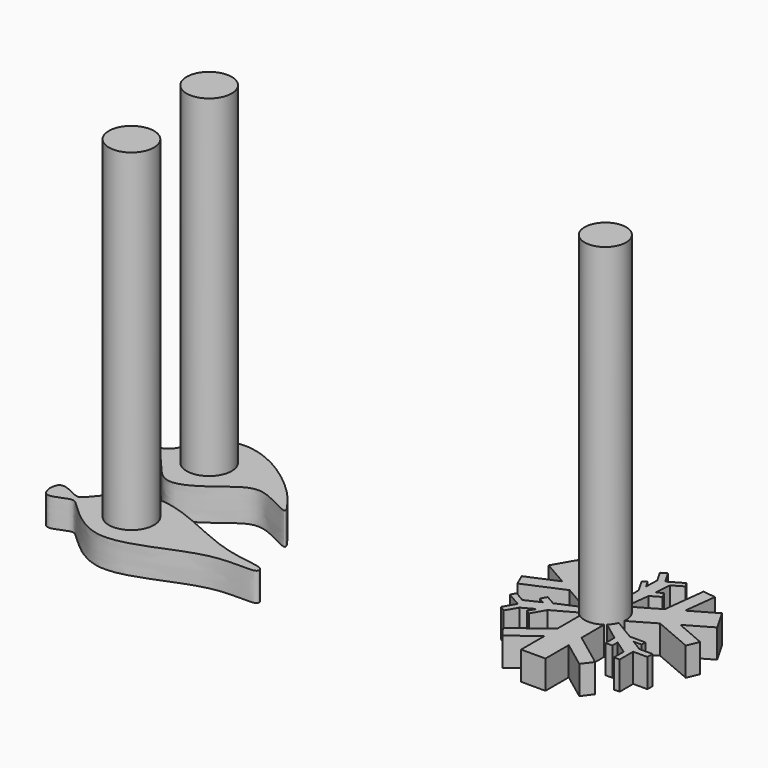
from build123d import *

# Parameters (mm, degrees)
F2_DEPTH  = 2
F1_R      = 1.4605
F3_DEPTH  = 25.4
F5_DEPTH  = 1
F7_SCALE  = 2.25
F9_R      = 1.5875
F10_DEPTH = 25.4
F13_DEPTH = 2
F12_R     = 1.5875
F14_DEPTH = 25.4


# Not quite as in the source:
# - ends of sketch curves that miss each other by under 0.0002 mm in the source are joined
# - a feature names something its author has since deleted; it is built from what else it names


with BuildPart() as f2:
    # F0 (on Top) → F2 (new body)
    with BuildSketch(Plane.XY):
        Polygon((0.3471141813, -0.6012196677), (-0.1371353539, -0.2375256701), (-0.2495522491, -0.4322374442), (-0.4318002417, -0.747900227), (-0.6211034032, -0.6386059958), (-0.8508992831, -0.7662402189), (-0.8508992831, -3.1749998652), (-0.8508992831, -4.3027643429), (-0.8508992831, -6.3499998652), (0.8636007169, -6.3499998652), (0.8636007169, -4.3027643429), (0.8636007169, -3.1749998652), (0.8636007169, -0.9891251569), (0.483299174, -0.703500952), (0.4254495248, -0.7369004626), align=None)
        Polygon((-0.8508992831, -4.3027643429), (-0.8508992831, -3.1749998652), (-3.2412230885, -4.9631580294), (-2.7002857532, -5.6862570345), align=None)
        Polygon((3.2539245223, -4.9631580294), (0.8636007169, -3.1749998652), (0.8636007169, -4.3027643429), (2.7129871871, -5.6862570345), align=None)
        Polygon((-0.8508992831, -0.0667988863), (-0.6942285962, 1.348e-07), (-0.8508992831, 1.348e-07), align=None)
        Polygon((-0.6942285962, 1.348e-07), (-0.1371355874, 0.2375255353), (-0.2495524826, 0.4322373094), (-0.4318004752, 0.7479000922), (-0.2424973138, 0.8571943234), (-0.2381338534, 1.1200205046), (-2.3241808987, 2.3244003278), (-3.3008535859, 2.8882825667), (-5.0738115558, 3.9119003278), (-5.9310615558, 2.427099773), (-4.1581035859, 1.4034820119), (-3.1814308987, 0.839599773), (-1.2884078719, -0.2533375811), (-0.8508992831, -0.0667988863), (-0.8508992831, 1.348e-07), align=None)
        Polygon((-0.8508992831, -0.7662402189), (-0.8508992831, -0.5059332827), (-1.2884078719, -0.2533375811), (-2.9236705151, -0.950557629), (-3.6042041051, -0.5576513776), (-3.8423290847, -0.9700959409), (-3.4298843198, -1.208221037), (-4.4835569455, -1.6997353006), (-5.2259572804, -1.2711102674), (-5.4283635946, -1.6216882874), (-4.3972519847, -2.2170008529), (-4.8973144653, -3.0831344762), (-4.5054921503, -3.3093531953), (-4.0411482187, -2.5050859137), (-3.2032690115, -2.0539615173), (-3.4890190337, -2.5488950739), (-3.2003078595, -2.7155825481), (-2.6526203364, -1.7669599314), align=None)
        Polygon((-5.9251831976, -0.3364022836), (-3.1814308987, 0.839599773), (-4.1581035859, 1.4034820119), (-6.2809366379, 0.4936126931), align=None)
        Polygon((-3.3008535859, 2.8882825667), (-2.3241808987, 2.3244003278), (-2.6776093922, 5.2885605486), (-3.5743001677, 5.181644577), align=None)
        Polygon((-0.0127014339, 0.9898670365), (0.4248071549, 1.242462738), (0.6386282031, 3.0072517529), (1.3191617931, 3.4001580042), (1.0810368134, 3.8126025675), (0.6685920485, 3.5744774715), (0.7697645227, 4.7327418644), (1.5121648577, 5.1613668976), (1.3097585434, 5.5119449176), (0.2786469335, 4.916632352), (-0.2214155471, 5.7827659754), (-0.6132378621, 5.5565472563), (-0.1488939305, 4.7522799747), (-0.1771483466, 3.8010930978), (-0.4628983688, 4.2960266544), (-0.7516095429, 4.1293391803), (-0.2039220199, 3.1807165637), (-0.2381338534, 1.1200205046), align=None)
        Polygon((2.6712586753, 5.299560313), (2.3178301818, 2.3354000922), (3.294502869, 2.8992823311), (3.5679494508, 5.1926443415), align=None)
        Polygon((0.2742709413, 1.348e-07), (0.4991047317, 1.348e-07), (0.8636007169, 1.348e-07), (0.8636007169, -0.2185883276), (1.0890331365, -0.3537802858), (3.1750801818, 0.8505995374), (4.151752869, 1.4144817763), (5.9247108388, 2.4380995374), (5.0674608388, 3.9229000922), (3.294502869, 2.8992823311), (2.3178301818, 2.3354000922), (0.4248071549, 1.242462738), (0.3676001091, 0.7702998383), (0.4254497583, 0.7369003278), (0.3471144148, 0.6012195329), align=None)
        Polygon((4.151752869, 1.4144817763), (3.1750801818, 0.8505995374), (5.9188324807, -0.3254025192), (6.274585921, 0.5046124575), align=None)
        Polygon((1.0890331365, -0.3537802858), (0.8636007169, -0.4839337539), (0.8636007169, -0.9891251569), (2.285042312, -2.0566941239), (2.285042312, -2.8425066266), (2.7612922713, -2.8425066266), (2.7612922713, -2.3662564345), (3.7137924228, -3.0330065638), (3.7137924228, -3.8902566303), (4.1186050512, -3.8902566303), (4.1186050512, -2.6996314991), (5.1187300123, -2.6996314991), (5.1187300123, -2.2471940611), (4.1900421493, -2.2471940611), (3.3804173581, -1.7471315805), (3.9519174024, -1.7471315805), (3.9519174024, -1.4137566322), (2.8565423563, -1.4137566322), align=None)
        Polygon((0.8636007169, -0.2185883276), (0.4991047317, 1.348e-07), (0.2742709413, 1.348e-07), (0.2266974185, -0.3926517164), (0.3471141813, -0.6012196677), (0.483299174, -0.703500952), (0.8636007169, -0.4839337539), align=None)
        Polygon((-0.1371353539, -0.2375256701), (-0.4533950705, 1.348e-07), (-0.6942285962, 1.348e-07), (-0.8508992831, -0.0667988863), (-0.8508992831, -0.5059332827), (-0.6211034032, -0.6386059958), (-0.2495522491, -0.4322374442), align=None)
        Polygon((0.226697652, 0.3926515816), (0.3471144148, 0.6012195329), (0.3676001091, 0.7702998383), (-0.0127014339, 0.9898670365), (-0.2424973138, 0.8571943234), (-0.2495524826, 0.4322373094), (-0.1371355874, 0.2375255353), align=None)
        Polygon((-0.0127014339, 0.9898670365), (0.3676001091, 0.7702998383), (0.4248071549, 1.242462738), align=None)
        Polygon((1.0890331365, -0.3537802858), (0.8636007169, -0.2185883276), (0.8636007169, -0.4839337539), align=None)
        Polygon((-0.4318002417, -0.747900227), (-0.2495522491, -0.4322374442), (-0.6211034032, -0.6386059958), align=None)
        Polygon((-0.8508992831, -0.7662402189), (-0.6211034032, -0.6386059958), (-0.8508992831, -0.5059332827), align=None)
        Polygon((-0.4318004752, 0.7479000922), (-0.2495524826, 0.4322373094), (-0.2424973138, 0.8571943234), align=None)
        Polygon((-0.2424973138, 0.8571943234), (-0.0127014339, 0.9898670365), (-0.2381338534, 1.1200205046), align=None)
        Polygon((0, 1.348e-07), (0.2742709413, 1.348e-07), (0.3471144148, 0.6012195329), (0.226697652, 0.3926515816), align=None)
        Polygon((-0.1371355874, 0.2375255353), (-1.167e-07, -6.74e-08), (0.226697652, 0.3926515816), align=None)
        Polygon((-0.4533950705, 1.348e-07), (0, 1.348e-07), (-0.1371355874, 0.2375255353), (-0.6942285962, 1.348e-07), align=None)
        Polygon((-0.1371353539, -0.2375256701), (1.167e-07, -6.74e-08), (-0.4533950705, 1.348e-07), align=None)
        Polygon((0.2266974185, -0.3926517164), (-1.167e-07, -6.74e-08), (-0.1371353539, -0.2375256701), (0.3471141813, -0.6012196677), align=None)
        Polygon((0.2266974185, -0.3926517164), (0.2742709413, 1.348e-07), (0, 1.348e-07), align=None)
        Polygon((0.3676001091, 0.7702998383), (0.3471144148, 0.6012195329), (0.4254497583, 0.7369003278), align=None)
        Polygon((0.483299174, -0.703500952), (0.3471141813, -0.6012196677), (0.4254495248, -0.7369004626), align=None)
    extrude(amount=F2_DEPTH)

    # F1 (on Top) → F3 (join)
    with BuildSketch(Plane.XY):
        Circle(F1_R)
    extrude(amount=F3_DEPTH)


with BuildPart() as f5:
    # F4 (on Top) → F5 (new body)
    with BuildSketch(Plane.XY):
        with BuildLine():
            add(Edge.make_bspline(
                [(-29.8669375479, 0.2857499931), (-29.7440304745, 0.3571436979), (-29.1547614666, -0.031081706), (-28.6573535606, 1.9086215428), (-26.8097076406, 1.4876465764), (-25.6137182394, 0.4424417951), (-25.3000873709, 0.0757578444), (-24.7765698555, -0.6160305024), (-25.5747691832, -0.1631625611), (-26.2801418295, 0.1338939544), (-26.9852315195, -0.4157522042), (-28.4156101147, -1.4829106615), (-29.1578723902, 0.3232844338), (-30.049192476, -0.1925589818), (-29.9590967439, 0.2322169762), (-29.8669375479, 0.2857499931)],
                knots=[0, 0, 0, 0, 0.0595602967, 0.1590621278, 0.2623182491, 0.3653254409, 0.4276419031, 0.4859643703, 0.5478739218, 0.6200200353, 0.696962825, 0.7939279281, 0.8918484857, 0.9553400069, 1, 1, 1, 1], degree=3))
        make_face()
    extrude(amount=F5_DEPTH)


with BuildPart() as f5_1:
    # F7: moved
    add(f5.part.scale(F7_SCALE).moved(Location((34.892889671, -0.5655468703, -1.25))))


with BuildPart() as f5_2:
    # F8: moved
    add(f5_1.part.moved(Location((0, 0, 1))))

    # F9 (on Top) → F10 (join)
    with BuildSketch(Plane.XY):
        with Locations((-28.1345900148, 0.302218803)):
            Circle(F9_R)
    extrude(amount=F10_DEPTH)


with BuildPart() as f13:
    # F11 (on Top) → F13 (new body)
    with BuildSketch(Plane.XY):
        with BuildLine():
            add(Edge.make_bspline(
                [(-32.8794009984, -6.9053298794), (-32.5540037989, -6.6793889467), (-31.3817308567, -7.5046151757), (-30.8072401032, -7.2022586946), (-28.1363850092, -3.1875440328), (-21.5654529107, -7.6163391855), (-17.9706751628, -7.4839443562), (-17.9570012573, -8.4361565431), (-21.5566094546, -7.6507221771), (-27.4242880142, -11.6673001261), (-30.7065035244, -8.0803469893), (-31.3631183292, -7.6668234126), (-33.0996125613, -8.8138189541), (-33.1778014741, -7.1125255219), (-32.8794009984, -6.9053298794)],
                knots=[0, 0, 0, 0, 0.0668292197, 0.1079970099, 0.2106914958, 0.3585719071, 0.4553176788, 0.4852046131, 0.5798662681, 0.721373447, 0.8281432135, 0.8738706847, 0.9387152963, 1, 1, 1, 1], degree=3))
        make_face()
    extrude(amount=F13_DEPTH)

    # F12 (on Top) → F14 (join)
    with BuildSketch(Plane.XY):
        with Locations((-27.4518691003, -7.3880827986)):
            Circle(F12_R)
    extrude(amount=F14_DEPTH)


solid = Compound([f2.part, f5_2.part, f13.part])
